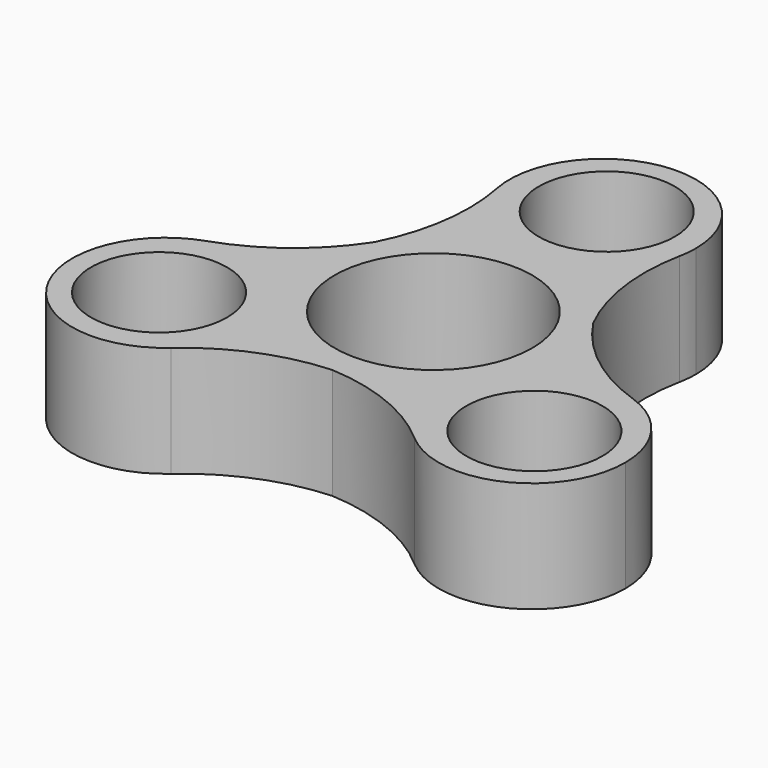
from build123d import *

# Parameters (mm, degrees)
F0_R        = 1.7145
F0_R_2      = 2.4892
F1_DEPTH    = 2.794
F2_T1_DEPTH = 2.794


# Not quite as in the source:
# - a fillet or chamfer that OpenCascade refuses, or shapes differently, is made with other operations: its cross-section is extruded or revolved along the edge and cut away or added
# - a feature names something its author has since deleted; it is built from what else it names


with BuildPart() as f1:
    # F0 (on Top) → F1 (new body)
    with BuildSketch(Plane.XY):
        with BuildLine():
            ThreePointArc((-2.2698795038, -2.667), (-2.7244789735, -1.2779347638), (-3.9123585253, -0.4264037432))
            ThreePointArc((-3.9123585253, -0.4264037432), (-6.65410619, -3.84175), (-2.3254557365, -3.175))
            ThreePointArc((-2.3254557365, -3.175), (-2.2838148888, -2.922515517), (-2.2698795038, -2.667))
        make_face()
        with Locations((-4.7293647301, -2.7305)):
            Circle(F0_R, mode=Mode.SUBTRACT)
        with BuildLine():
            ThreePointArc((6.9688795038, -2.667), (6.00844474, -0.7720994698), (3.9123585253, -0.4264037432))
            ThreePointArc((3.9123585253, -0.4264037432), (2.5846528176, -1.49225), (2.3254557365, -3.175))
            ThreePointArc((2.3254557365, -3.175), (4.8748950208, -5.0025646149), (6.9688795038, -2.667))
        make_face()
        with Locations((4.7293647301, -2.7305)):
            Circle(F0_R, mode=Mode.SUBTRACT)
        with BuildLine():
            ThreePointArc((1.5869027888, 3.6014037432), (2.1504160472, 4.3875006213), (2.3495, 5.334))
            ThreePointArc((2.3495, 5.334), (-0.9464993787, 7.4844160472), (-1.5869027888, 3.6014037432))
            ThreePointArc((-1.5869027888, 3.6014037432), (0, 2.9845), (1.5869027888, 3.6014037432))
        make_face()
        with Locations((0, 5.461)):
            Circle(F0_R, mode=Mode.SUBTRACT)
        with BuildLine():
            ThreePointArc((1.5869027888, 3.6014037432), (0, 2.9845), (-1.5869027888, 3.6014037432))
            Line((-1.5869027888, 3.6014037432), (-3.9123585253, -0.4264037432))
            ThreePointArc((-3.9123585253, -0.4264037432), (-2.7244789735, -1.2779347638), (-2.2698795038, -2.667))
            ThreePointArc((-2.2698795038, -2.667), (-2.2838148888, -2.922515517), (-2.3254557365, -3.175))
            Line((-2.3254557365, -3.175), (2.3254557365, -3.175))
            ThreePointArc((2.3254557365, -3.175), (2.5846528176, -1.49225), (3.9123585253, -0.4264037432))
            Line((3.9123585253, -0.4264037432), (1.5869027888, 3.6014037432))
        make_face()
        Circle(F0_R_2, mode=Mode.SUBTRACT)
    extrude(amount=F1_DEPTH)

    # F2: fillet of radius 5.08 on 6 edges, made by hand

    # F2_s2 → F2_t1 (join)
    with BuildSketch(Plane.XY):
        with BuildLine():
            ThreePointArc((-5.3756036804, -0.4425280976), (-3.7870806895, 0.4409737593), (-2.6112739301, 1.8271408806))
            Line((-2.6112739301, 1.8271408806), (-3.9123585253, -0.4264037432))
            ThreePointArc((-3.9123585253, -0.4264037432), (-4.6452684469, -0.3176426384), (-5.3756036804, -0.4425280976))
        make_face()
        with BuildLine():
            ThreePointArc((-3.0710424146, -4.4341452991), (-1.5116458668, -3.500194963), (0.2767134539, -3.175))
            Line((0.2767134539, -3.175), (-2.3254557365, -3.175))
            ThreePointArc((-2.3254557365, -3.175), (-2.5977208176, -3.8640991633), (-3.0710424146, -4.4341452991))
        make_face()
        with BuildLine():
            ThreePointArc((5.3756036804, -0.4425280976), (3.7870806895, 0.4409737593), (2.6112739301, 1.8271408806))
            Line((2.6112739301, 1.8271408806), (3.9123585253, -0.4264037432))
            ThreePointArc((3.9123585253, -0.4264037432), (4.6452684469, -0.3176426384), (5.3756036804, -0.4425280976))
        make_face()
        with BuildLine():
            ThreePointArc((-0.2767134539, -3.175), (1.5116458668, -3.500194963), (3.0710424146, -4.4341452991))
            ThreePointArc((3.0710424146, -4.4341452991), (2.5977208176, -3.8640991633), (2.3254557365, -3.175))
            Line((2.3254557365, -3.175), (-0.2767134539, -3.175))
        make_face()
        with BuildLine():
            ThreePointArc((2.887987384, 1.3478591194), (2.2754348227, 3.0592212037), (2.3045612658, 4.8766733967))
            ThreePointArc((2.3045612658, 4.8766733967), (2.0475476293, 4.1817418016), (1.5869027888, 3.6014037432))
            Line((1.5869027888, 3.6014037432), (2.887987384, 1.3478591194))
        make_face()
        with BuildLine():
            ThreePointArc((-2.3045612658, 4.8766733967), (-2.2754348227, 3.0592212037), (-2.887987384, 1.3478591194))
            Line((-2.887987384, 1.3478591194), (-1.5869027888, 3.6014037432))
            ThreePointArc((-1.5869027888, 3.6014037432), (-2.0475476293, 4.1817418016), (-2.3045612658, 4.8766733967))
        make_face()
    extrude(amount=F2_T1_DEPTH)


solid = f1.part
